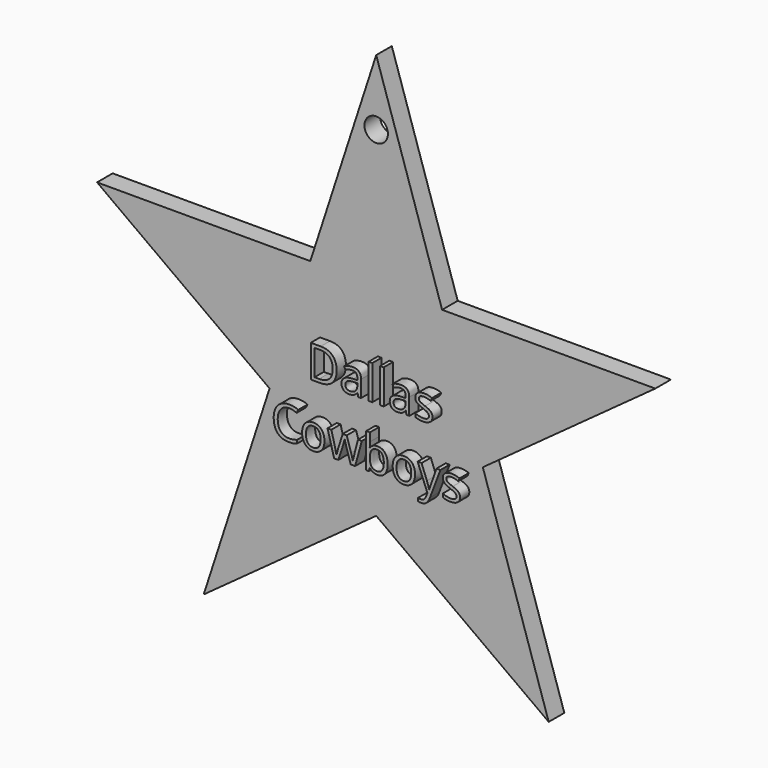
from build123d import *

# Parameters (mm, degrees)
F0_R         = 4.2830449481
F1_DEPTH     = 7.112
F2_TEXT_SIZE = 16.56501942
F3_DEPTH     = 4.2164


# Not quite as in the source:
# - Text() gives the source's letters only with a copy of the font that has no kerning and outlines rounded to 1/6400 em; it was checked with that copy


with BuildPart() as f1:
    # F0 (on Front) → F1 (new body)
    with BuildSketch(Plane.XZ):
        Polygon((-62.9281162645, -86.6131215158), (0, -40.8931688423), (62.9281162645, -86.6131215158), (38.8917146995, -12.6366841261), (101.819830964, 33.0832685473), (24.036401565, 33.0832685473), (0, 107.0597059369), (-24.036401565, 33.0832685473), (-101.819830964, 33.0832685473), (-38.8917146995, -12.6366841261), align=None)
        Polygon((-25.7535387788, -8.3678319969), (-67.4236398534, 21.9072685801), (-15.9165622959, 21.9072685801), (0, 70.8934103265), (15.9165622959, 21.9072685801), (67.4236398534, 21.9072685801), (25.7535387788, -8.3678319969), (41.6701010746, -57.3539737433), (0, -27.0788731663), (-41.6701010746, -57.3539737433), align=None, mode=Mode.SUBTRACT)
        with Locations((0, 83.1125378609)):
            Circle(F0_R, mode=Mode.SUBTRACT)
        Polygon((-15.9165622959, 21.9072685801), (-67.4236398534, 21.9072685801), (-25.7535387788, -8.3678319969), (-41.6701010746, -57.3539737433), (0, -27.0788731663), (41.6701010746, -57.3539737433), (25.7535387788, -8.3678319969), (67.4236398534, 21.9072685801), (15.9165622959, 21.9072685801), (0, 70.8934103265), align=None)
    extrude(amount=-F1_DEPTH)

    # F2 (on face) → F3 (join)
    with BuildSketch(Plane.XZ):
        with Locations((-22.1181833522, -2.0864785183)):
            Text('Dallas', F2_TEXT_SIZE, font='Open Sans', text_align=(TextAlign.LEFT, TextAlign.BOTTOM))
        with Locations((-35.031133647, -24.6149049296)):
            Text('Cowboys', F2_TEXT_SIZE, font='Open Sans', text_align=(TextAlign.LEFT, TextAlign.BOTTOM))
    extrude(amount=F3_DEPTH)


solid = f1.part
